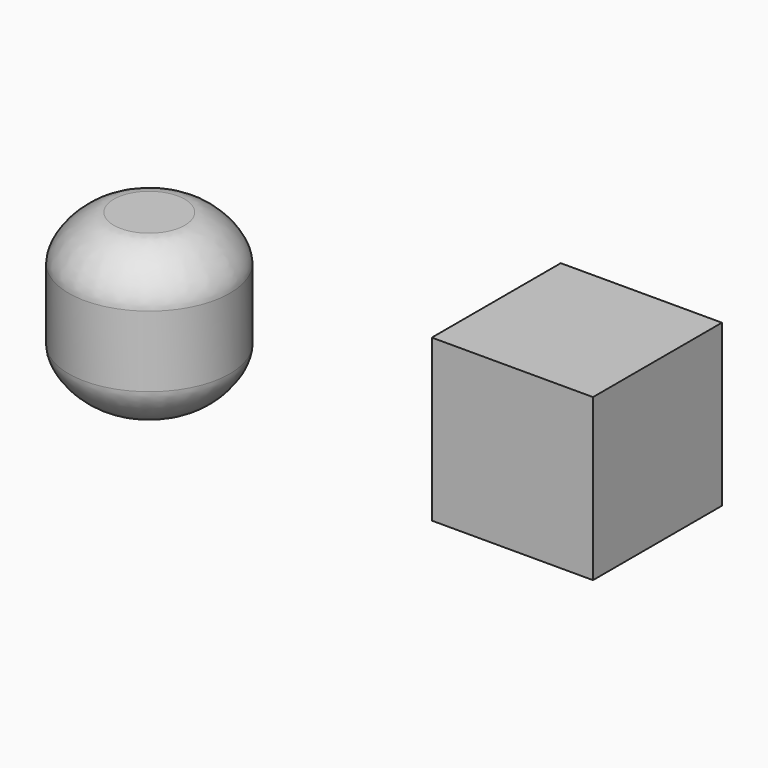
from build123d import *

# Parameters (mm, degrees)
F0_W     = 25
F0_H     = 25
F1_DEPTH = 25
F2_R     = 12.5
F3_DEPTH = 25


# Not quite as in the source:
# - a fillet or chamfer that OpenCascade refuses, or shapes differently, is made with other operations: its cross-section is extruded or revolved along the edge and cut away or added


with BuildPart() as f1:
    # F0 (on Front) → F1 (new body)
    with BuildSketch(Plane.XZ):
        with Locations((12.5, 12.5)):
            Rectangle(F0_W, F0_H)
    extrude(amount=F1_DEPTH)


with BuildPart() as f3:
    # F2 (on Top) → F3 (new body)
    with BuildSketch(Plane.XY):
        with Locations((-47.2602769732, -20.7147393376)):
            Circle(F2_R)
    extrude(amount=F3_DEPTH)

    # F4: fillet of radius 7 on 2 edges, made by hand

    # F4_s1 → F4_t2 (revolve, cut)
    with BuildSketch(Plane.XZ.offset(20.7147393376)):
        with BuildLine():
            add(Edge.make_bspline(
                [(-34.7602769732, 18), (-34.7602769732, 25), (-41.7602769732, 25)],
                knots=[0, 0, 0, 1, 1, 1], degree=2, weights=[1, 0.4285714286, 1]))
            Line((-41.7602769732, 25), (-34.7602769732, 25))
            Line((-34.7602769732, 25), (-34.7602769732, 18))
        make_face()
    revolve(axis=Axis((-47.2602769732, -20.7147393376, 25), (0, 0, 1)), mode=Mode.SUBTRACT)

    # F4_s3 → F4_t4 (revolve, cut)
    with BuildSketch(Plane.XZ.offset(20.7147393376)):
        with BuildLine():
            add(Edge.make_bspline(
                [(-34.7602769732, 7), (-34.7602769732, 0), (-41.7602769732, 0)],
                knots=[0, 0, 0, 1, 1, 1], degree=2, weights=[1, 0.4285714286, 1]))
            Line((-41.7602769732, 0), (-34.7602769732, 0))
            Line((-34.7602769732, 0), (-34.7602769732, 7))
        make_face()
    revolve(axis=Axis((-47.2602769732, -20.7147393376, 0), (0, 0, 1)), mode=Mode.SUBTRACT)


solid = Compound([f1.part, f3.part])
